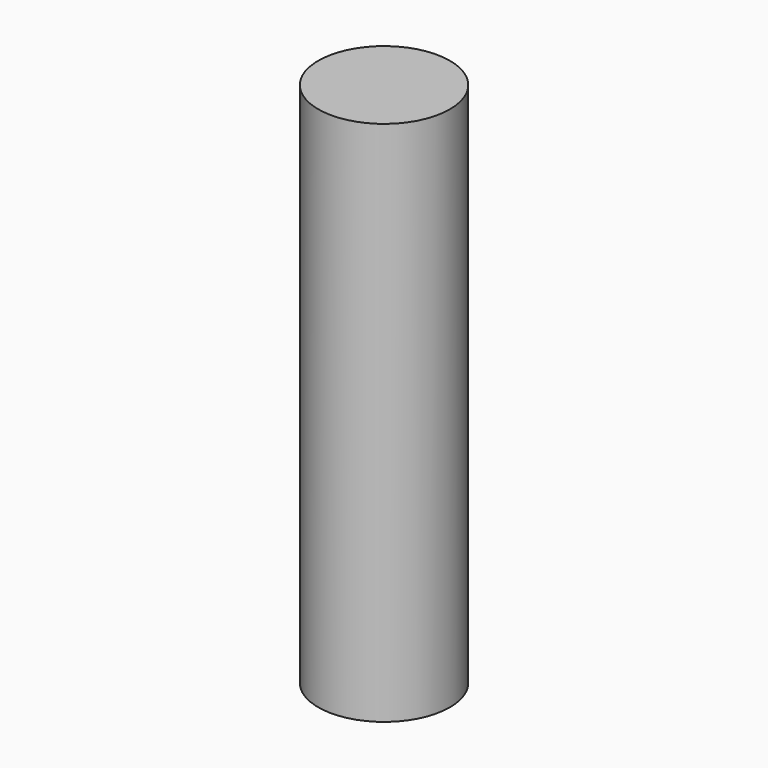
from build123d import *


# Not quite as in the source:
# - the program builds the solid bodies; features that only make, move or delete a surface that nothing else refers to are left out


with BuildPart() as f2:
    # F0 (on Front) → F2 (revolve)
    with BuildSketch(Plane.XZ):
        with BuildLine():
            Line((-6.25, -50), (6.25, -50))
            Line((6.25, -50), (6.25, 50))
            Line((6.25, 50), (-6.25, 50))
            Line((-6.25, 50), (-6.25, 39.189))
            ThreePointArc((-6.25, 39.189), (-5.0556966466, 38.6943033534), (-4.561, 37.5))
            ThreePointArc((-4.561, 37.5), (-5.0556966466, 36.3056966466), (-6.25, 35.811))
            Line((-6.25, 35.811), (-6.25, -50))
        make_face()
        with BuildLine():
            ThreePointArc((-6.25, 39.189), (-7.939, 37.5), (-6.25, 35.811))
            Line((-6.25, 35.811), (-6.25, 39.189))
        make_face()
        with BuildLine():
            Line((-6.25, 39.189), (-6.25, 35.811))
            ThreePointArc((-6.25, 35.811), (-5.0556966466, 36.3056966466), (-4.561, 37.5))
            ThreePointArc((-4.561, 37.5), (-5.0556966466, 38.6943033534), (-6.25, 39.189))
        make_face()
    revolve(axis=Axis((-6.25, 0, 0), (0, 0, 1)))


solid = f2.part
